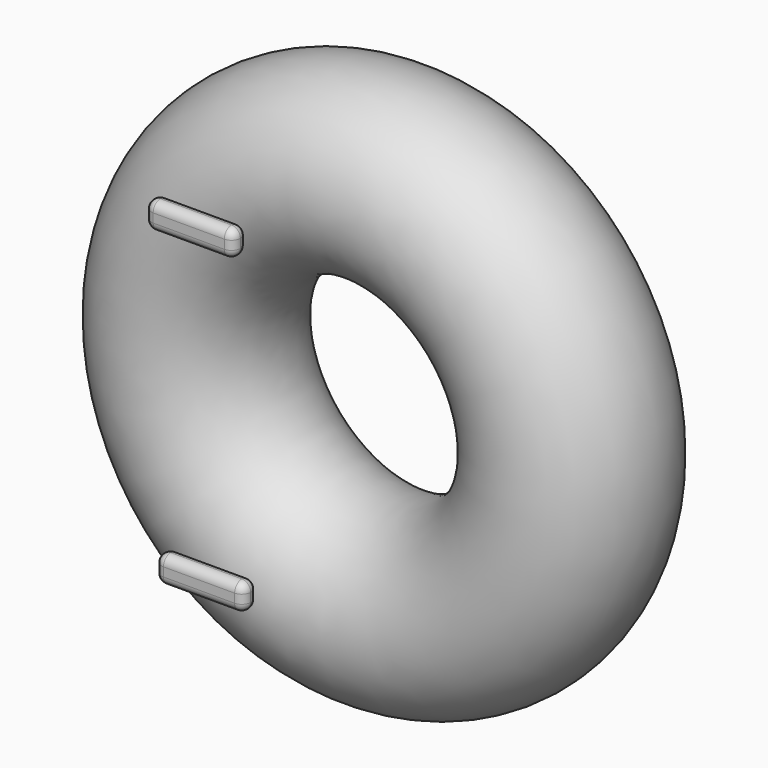
from build123d import *

# Parameters (mm, degrees)
F0_R     = 50
F3_W     = 50
F3_H     = 15
F4_DEPTH = 10
F5_R     = 4.99999


# Not quite as in the source:
# - a fillet or chamfer is up to 0.001 mm smaller than in the source, because OpenCascade refuses the exact size


with BuildPart() as f1:
    # F0 (on Top) → F1 (revolve)
    with BuildSketch(Plane.XY):
        Circle(F0_R)
    revolve(axis=Axis((-105.4752663247, 0.8680145796, 0), (0, -1, 0)))


with BuildPart() as f4:
    # F3 (on offset) → F4 (new body)
    with BuildSketch(Plane.XZ.offset(50)):
        with Locations((-167.2578901052, 79.9979186445)):
            Rectangle(F3_W, F3_H)
    extrude(amount=F4_DEPTH)

    # F5 (radius 5 in the source; OpenCascade refuses exactly that, so slightly less here)
    f5_edges = [f4.edges().sort_by_distance(p)[0] for p in [
        (-192.25789, -60, 79.997919),
        (-142.25789, -55, 87.497919),
        (-192.25789, -55, 87.497919),
        (-167.25789, -50, 87.497919),
        (-167.25789, -60, 87.497919),
        (-167.25789, -60, 72.497919),
        (-142.25789, -60, 79.997919),
        (-192.25789, -55, 72.497919),
        (-192.25789, -50, 79.997919),
        (-142.25789, -55, 72.497919),
        (-167.25789, -50, 72.497919),
        (-142.25789, -50, 79.997919),
    ]]
    fillet(f5_edges, radius=F5_R)


with BuildPart() as f6_1:
    # F6: copy of F4
    add(f4.part.moved(Location((5, 1, -174))))


solid = Compound([f1.part, f4.part, f6_1.part])
